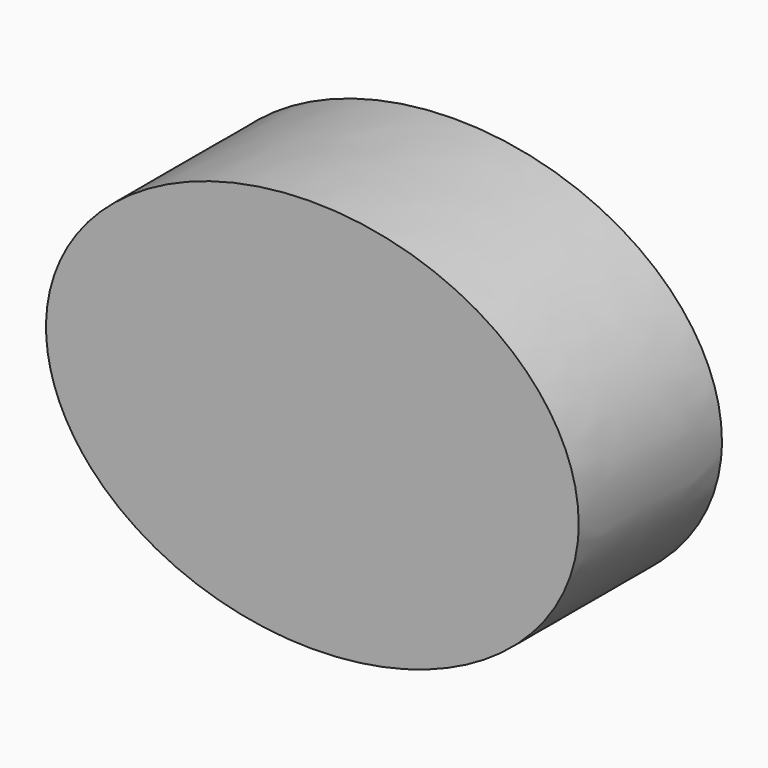
from build123d import *

# Parameters (mm, degrees)
F3_DEPTH = 25.4
F2_R     = 5.328555548
F4_DEPTH = 25.4


# Not quite as in the source:
# - the program builds the solid bodies; features that only make, move or delete a surface that nothing else refers to are left out


with BuildPart() as f3:
    # F0 (on Front) → F3 (new body)
    with BuildSketch(Plane.XZ):
        with BuildLine():
            add(Edge.make_bspline(
                [(37.7864688635, 0), (37.7864688635, 48.3628191549), (-18.8932344317, 24.1814095774), (-75.572937727, 0), (-18.8932344317, -24.1814095774), (37.7864688635, -48.3628191549), (37.7864688635, 0)],
                knots=[0, 0, 0, 2.0943951024, 2.0943951024, 4.1887902048, 4.1887902048, 6.2831853072, 6.2831853072, 6.2831853072], degree=2, weights=[1, 0.5, 1, 0.5, 1, 0.5, 1]))
        make_face()
    extrude(amount=F3_DEPTH)

    # F2 (on face) → F4 (cut)
    with BuildSketch(Plane.XZ):
        Circle(F2_R)
    extrude(amount=-F4_DEPTH, mode=Mode.SUBTRACT)


solid = f3.part
